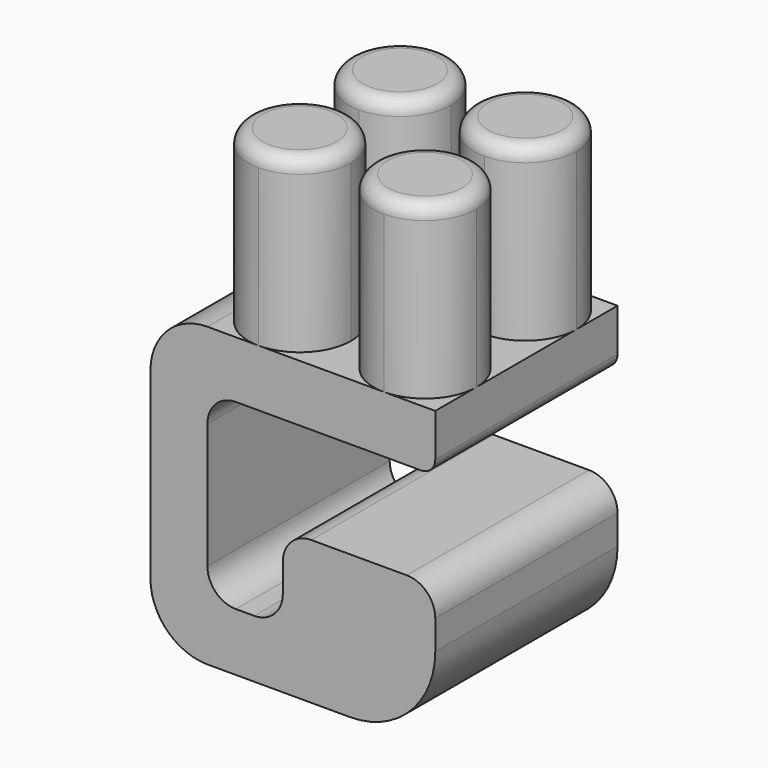
from build123d import *

# Parameters (mm, degrees)
F1_DEPTH = 20
F3_DEPTH = 30


# Not quite as in the source:
# - a fillet or chamfer that OpenCascade refuses, or shapes differently, is made with other operations: its cross-section is extruded or revolved along the edge and cut away or added
# - a feature names something its author has since deleted; it is built from what else it names


with BuildPart() as f1:
    # F0 (on Front) → F1 (new body, symmetric)
    with BuildSketch(Plane.XZ):
        with BuildLine():
            Line((-10, -5), (17.5, -5))
            ThreePointArc((17.5, -5), (19.267766953, -4.267766953), (20, -2.5))
            Line((20, -2.5), (20, 5))
            Line((20, 5), (-20, 5))
            ThreePointArc((-20, 5), (-27.0710678119, 2.0710678119), (-30, -5))
            Line((-30, -5), (-30, -37.0084848255))
            Line((-30, -37.0084848255), (-29.9999700785, -37.1900333921))
            ThreePointArc((-29.9999700785, -37.1900333921), (-27.134358967, -44.1955599538), (-20.1815186475, -47.1867371371))
            Line((-20.1815186475, -47.1867371371), (-20, -47.1900331229))
            Line((-20, -47.1900331229), (-10, -47.1900331229))
            Line((-10, -47.1900331229), (-6.8265195005, -47.1900331229))
            Line((-6.8265195005, -47.1900331229), (5, -47.1900331229))
            ThreePointArc((5, -47.1900331229), (15.6066017178, -42.7966348407), (20, -32.1900331229))
            Line((20, -32.1900331229), (20, -32.0304483175))
            Line((20, -32.0304483175), (20, -27.0304483175))
            ThreePointArc((20, -27.0304483175), (18.5355339059, -23.4949144116), (15, -22.0304483175))
            Line((15, -22.0304483175), (3.1734804995, -22.0304483175))
            Line((3.1734804995, -22.0304483175), (-1.7689520504, -22.0304483175))
            ThreePointArc((-1.7689520504, -22.0304483175), (-5.3044859563, -23.4949144116), (-6.7689520504, -27.0304483175))
            Line((-6.7689520504, -27.0304483175), (-6.7689520504, -32.0304483175))
            ThreePointArc((-6.7689520504, -32.0304483175), (-8.2410406124, -35.5516728412), (-11.7686128262, -37.0084848255))
            Line((-11.7686128262, -37.0084848255), (-15, -37.0084848255))
            ThreePointArc((-15, -37.0084848255), (-18.5355339059, -35.5440187314), (-20, -32.0084848255))
            Line((-20, -32.0084848255), (-20, -15))
            Line((-20, -15), (-20, -10))
            ThreePointArc((-20, -10), (-18.5355339059, -6.4644660941), (-15, -5))
            Line((-15, -5), (-10, -5))
        make_face()
    extrude(amount=F1_DEPTH, both=True)

    # F2 (on face) → F3 (join)
    with BuildSketch(Plane.XY.offset(5)):
        with BuildLine():
            Line((-11, 11), (-2, 11))
            ThreePointArc((-2, 11), (-4.6360389693, 17.3639610307), (-11, 20))
            Line((-11, 20), (-11, 11))
        make_face()
        with BuildLine():
            Line((-20, 11), (-11, 11))
            Line((-11, 11), (-11, 20))
            ThreePointArc((-11, 20), (-17.3639610307, 17.3639610307), (-20, 11))
        make_face()
        with BuildLine():
            ThreePointArc((-20, 11), (-17.3639610288, 4.6360389675), (-10.9999999948, 2))
            Line((-11, 2), (-11, 11))
            Line((-11, 11), (-20, 11))
        make_face()
        with BuildLine():
            Line((-11, 11), (-11, 2))
            ThreePointArc((-10.9999999948, 2), (-4.6360389675, 4.6360389712), (-2, 11))
            Line((-2, 11), (-11, 11))
        make_face()
        with BuildLine():
            ThreePointArc((11, 20), (4.6360389693, 17.3639610307), (2, 11))
            Line((2, 11), (11, 11))
            Line((11, 11), (11, 20))
        make_face()
        with BuildLine():
            Line((11, 20), (11, 11))
            Line((11, 11), (20, 11))
            ThreePointArc((20, 11), (17.3639610307, 17.3639610307), (11, 20))
        make_face()
        with BuildLine():
            Line((11, 11), (11, 2))
            ThreePointArc((11, 2), (17.3639610307, 4.6360389693), (20, 11))
            Line((20, 11), (11, 11))
        make_face()
        with BuildLine():
            ThreePointArc((2, 11), (4.6360389693, 4.6360389693), (11, 2))
            Line((11, 2), (11, 11))
            Line((11, 11), (2, 11))
        make_face()
        with BuildLine():
            ThreePointArc((11, -2), (4.6360389693, -4.6360389693), (2, -11))
            Line((2, -11), (11, -11))
            Line((11, -11), (11, -2))
        make_face()
        with BuildLine():
            Line((11, -2), (11, -11))
            Line((11, -11), (20, -11))
            ThreePointArc((20, -11), (17.3639610307, -4.6360389693), (11, -2))
        make_face()
        with BuildLine():
            Line((11, -11), (11, -20))
            ThreePointArc((11, -20), (17.3639610307, -17.3639610307), (20, -11))
            Line((20, -11), (11, -11))
        make_face()
        with BuildLine():
            Line((11, -11), (2, -11))
            ThreePointArc((2, -11), (4.6360389693, -17.3639610307), (11, -20))
            Line((11, -20), (11, -11))
        make_face()
        with BuildLine():
            ThreePointArc((-11, -20), (-4.6360389693, -17.3639610307), (-2, -11))
            Line((-2, -11), (-11, -11))
            Line((-11, -11), (-11, -20))
        make_face()
        with BuildLine():
            ThreePointArc((-20, -11), (-17.3639610307, -17.3639610307), (-11, -20))
            Line((-11, -20), (-11, -11))
            Line((-11, -11), (-20, -11))
        make_face()
        with BuildLine():
            Line((-20, -11), (-11, -11))
            Line((-11, -11), (-11, -2))
            ThreePointArc((-11, -2), (-17.3639610307, -4.6360389693), (-20, -11))
        make_face()
        with BuildLine():
            Line((-11, -11), (-2, -11))
            ThreePointArc((-2, -11), (-4.6360389693, -4.6360389693), (-11, -2))
            Line((-11, -2), (-11, -11))
        make_face()
    extrude(amount=F3_DEPTH)

    # F4: fillet of radius 2.5 on 4 edges, made by hand

    # F4_s1 → F4_t2 (revolve, cut)
    with BuildSketch(Plane.YZ.offset(-11)):
        with BuildLine():
            ThreePointArc((2, 32.5), (2.732233047, 34.267766953), (4.5, 35))
            Line((4.5, 35), (2, 35))
            Line((2, 35), (2, 32.5))
        make_face()
    revolve(axis=Axis((-11, 11, 35), (0, 0, 1)), mode=Mode.SUBTRACT)

    # F4_s3 → F4_t4 (revolve, cut)
    with BuildSketch(Plane.XZ.offset(-11)):
        with BuildLine():
            ThreePointArc((2, 32.5), (2.732233047, 34.267766953), (4.5, 35))
            Line((4.5, 35), (2, 35))
            Line((2, 35), (2, 32.5))
        make_face()
    revolve(axis=Axis((11, 11, 35), (0, 0, 1)), mode=Mode.SUBTRACT)

    # F4_s5 → F4_t6 (revolve, cut)
    with BuildSketch(Plane.XZ.offset(11)):
        with BuildLine():
            ThreePointArc((2, 32.5), (2.732233047, 34.267766953), (4.5, 35))
            Line((4.5, 35), (2, 35))
            Line((2, 35), (2, 32.5))
        make_face()
    revolve(axis=Axis((11, -11, 35), (0, 0, 1)), mode=Mode.SUBTRACT)

    # F4_s7 → F4_t8 (revolve, cut)
    with BuildSketch(Plane.XZ.offset(11)):
        with BuildLine():
            ThreePointArc((-2, 32.5), (-2.732233047, 34.267766953), (-4.5, 35))
            Line((-4.5, 35), (-2, 35))
            Line((-2, 35), (-2, 32.5))
        make_face()
    revolve(axis=Axis((-11, -11, 35), (0, 0, 1)), mode=Mode.SUBTRACT)


solid = f1.part
